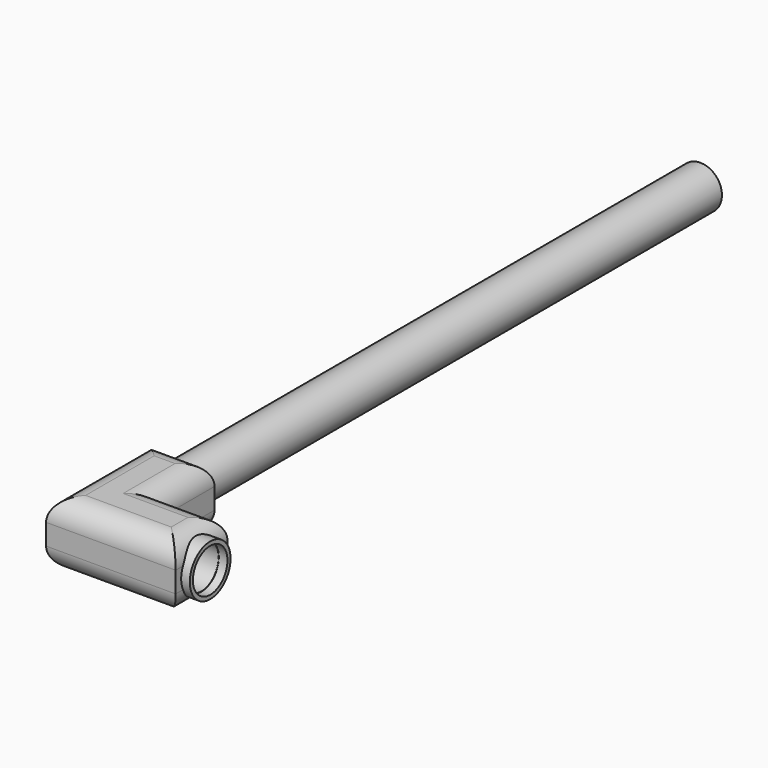
from build123d import *

# Parameters (mm, degrees)
F0_W          = 15
F0_H          = 15
F0_W_2        = 10
F0_H_2        = 10
F1_DEPTH      = 30
F2_W          = 15
F2_H          = 15
F2_W_2        = 10
F2_H_2        = 10
F4_DEPTH      = 15
F3_W          = 10
F3_H          = 10
F5_DEPTH      = 30
F6_R          = 5
F6_R_2        = 4.4707642424
F7_DEPTH      = 150
F8_W          = 10
F8_H          = 10
F9_DEPTH      = 15
F10_R         = 5.9
F10_R_2       = 5
F11_DEPTH     = 2
F12_R         = 4.929647133
F13_DEPTH     = 25.4
F14_T1_DEPTH  = 27.7
F14_T3_DEPTH  = 27.7
F14_T5_DEPTH  = 55.4
F14_T7_DEPTH  = 55.4
F14_T9_DEPTH  = 40.4
F14_T14_DEPTH = 40.4
F14_S15_R     = 5.9
F14_T16_DEPTH = 22
F14_T20_DEPTH = 40.4
F14_S21_R     = 5.9
F14_T22_DEPTH = 22
F14_T27_DEPTH = 27.7
F14_T31_DEPTH = 27.7
F14_S33_R     = 4.929647133
F14_T34_DEPTH = 16
F14_T40_DEPTH = 27.7
F14_T44_DEPTH = 27.7
F14_S46_R     = 4.929647133
F14_T47_DEPTH = 16


# Not quite as in the source:
# - a fillet or chamfer that OpenCascade refuses, or shapes differently, is made with other operations: its cross-section is extruded or revolved along the edge and cut away or added


with BuildPart() as f1:
    # F0 (on Front) → F1 (new body)
    with BuildSketch(Plane.XZ):
        Rectangle(F0_W, F0_H)
        Rectangle(F0_W_2, F0_H_2, mode=Mode.SUBTRACT)
    extrude(amount=F1_DEPTH)

    # F2 (on face) → F4 (join)
    with BuildSketch(Plane.YZ.offset(7.5)):
        with Locations((-22.5, 0)):
            Rectangle(F2_W, F2_H)
        with Locations((-22.5, 0)):
            Rectangle(F2_W_2, F2_H_2, mode=Mode.SUBTRACT)
    extrude(amount=F4_DEPTH)

    # F3 (on face) → F5 (join)
    with BuildSketch(Plane.XZ.offset(30)):
        Rectangle(F3_W, F3_H)
    extrude(amount=-F5_DEPTH)

    # F8 (on face) → F9 (join)
    with BuildSketch(Plane.YZ.offset(7.5)):
        with Locations((-22.5, 0)):
            Rectangle(F8_W, F8_H)
    extrude(amount=F9_DEPTH)

    # F10 (on face) → F11 (join)
    with BuildSketch(Plane.YZ.offset(22.5)):
        with Locations((-22.5, 0)):
            Circle(F10_R)
        with Locations((-22.5, 0)):
            Circle(F10_R_2, mode=Mode.SUBTRACT)
    extrude(amount=F11_DEPTH)

    # F12 (on face) → F13 (cut)
    with BuildSketch(Plane.YZ.offset(22.5)):
        with Locations((-22.5, 0)):
            Circle(F12_R)
    extrude(amount=-F13_DEPTH, mode=Mode.SUBTRACT)

    # F14: fillet of radius 5.08 on 12 edges, made by hand

    # F14_s2 → F14_t1 (cut)
    with BuildSketch(Plane.XZ.offset(-12.7)):
        with BuildLine():
            ThreePointArc((7.5, 2.42), (6.0121024484, 6.0121024484), (2.42, 7.5))
            Line((2.42, 7.5), (7.5, 7.5))
            Line((7.5, 7.5), (7.5, 2.42))
        make_face()
        with BuildLine():
            ThreePointArc((2.42, -7.5), (6.0121024484, -6.0121024484), (7.5, -2.42))
            Line((7.5, -2.42), (7.5, -7.5))
            Line((7.5, -7.5), (2.42, -7.5))
        make_face()
    extrude(amount=F14_T1_DEPTH, mode=Mode.SUBTRACT)

    # F14_s4 → F14_t3 (cut)
    with BuildSketch(Plane.YZ.offset(7.5)):
        with BuildLine():
            ThreePointArc((-15, 2.42), (-16.4878975516, 6.0121024484), (-20.08, 7.5))
            Line((-20.08, 7.5), (-15, 7.5))
            Line((-15, 7.5), (-15, 2.42))
        make_face()
        with BuildLine():
            ThreePointArc((-20.08, -7.5), (-16.4878975516, -6.0121024484), (-15, -2.42))
            Line((-15, -2.42), (-15, -7.5))
            Line((-15, -7.5), (-20.08, -7.5))
        make_face()
    extrude(amount=F14_T3_DEPTH, mode=Mode.SUBTRACT)

    # F14_s6 → F14_t5 (cut)
    with BuildSketch(Plane.YZ.offset(-20.2)):
        with BuildLine():
            ThreePointArc((-30, 2.42), (-28.5121024484, 6.0121024484), (-24.92, 7.5))
            Line((-24.92, 7.5), (-30, 7.5))
            Line((-30, 7.5), (-30, 2.42))
        make_face()
        with BuildLine():
            ThreePointArc((-24.92, -7.5), (-28.5121024484, -6.0121024484), (-30, -2.42))
            Line((-30, -2.42), (-30, -7.5))
            Line((-30, -7.5), (-24.92, -7.5))
        make_face()
    extrude(amount=F14_T5_DEPTH, mode=Mode.SUBTRACT)

    # F14_s8 → F14_t7 (cut)
    with BuildSketch(Plane.XZ.offset(-12.7)):
        with BuildLine():
            ThreePointArc((-7.5, 2.42), (-6.0121024484, 6.0121024484), (-2.42, 7.5))
            Line((-2.42, 7.5), (-7.5, 7.5))
            Line((-7.5, 7.5), (-7.5, 2.42))
        make_face()
        with BuildLine():
            ThreePointArc((-2.42, -7.5), (-6.0121024484, -6.0121024484), (-7.5, -2.42))
            Line((-7.5, -2.42), (-7.5, -7.5))
            Line((-7.5, -7.5), (-2.42, -7.5))
        make_face()
    extrude(amount=F14_T7_DEPTH, mode=Mode.SUBTRACT)

    # F14_s10 → F14_t9 (cut)
    with BuildSketch(Plane.YZ.offset(-20.2)):
        with BuildLine():
            ThreePointArc((0, 2.42), (-1.4878975516, 6.0121024484), (-5.08, 7.5))
            Line((-5.08, 7.5), (0, 7.5))
            Line((0, 7.5), (0, 2.42))
        make_face()
        with BuildLine():
            ThreePointArc((-5.08, -7.5), (-1.4878975516, -6.0121024484), (0, -2.42))
            Line((0, -2.42), (0, -7.5))
            Line((0, -7.5), (-5.08, -7.5))
        make_face()
    extrude(amount=F14_T9_DEPTH, mode=Mode.SUBTRACT)


with BuildPart() as f7:
    # F6 (on face) → F7 (new body)
    with BuildSketch(Plane(origin=(0, 0, 0), x_dir=(-1, 0, 0), z_dir=(0, 1, 0))):
        Circle(F6_R)
        Circle(F6_R_2, mode=Mode.SUBTRACT)
    extrude(amount=F7_DEPTH)


with BuildPart() as f14_tool12:
    # F14_s13 → F14_t14 (new body)
    with BuildSketch(Plane.XZ.offset(2.3)):
        with BuildLine():
            ThreePointArc((22.5, 2.42), (21.0121024484, 6.0121024484), (17.42, 7.5))
            Line((17.42, 7.5), (22.5, 7.5))
            Line((22.5, 7.5), (22.5, 2.42))
        make_face()
    extrude(amount=F14_T14_DEPTH)

    # F14_s15 → F14_t16 (cut, symmetric)
    with BuildSketch(Plane.YZ.offset(20)):
        with Locations((-22.5, 0)):
            Circle(F14_S15_R)
    extrude(amount=F14_T16_DEPTH, both=True, mode=Mode.SUBTRACT)


with BuildPart() as f1_1:
    add(f1.part)

    # F14_t11: cut F14_tool12
    add(f14_tool12.part, mode=Mode.SUBTRACT)


with BuildPart() as f14_tool18:
    # F14_s19 → F14_t20 (new body)
    with BuildSketch(Plane.XZ.offset(42.7)):
        with BuildLine():
            ThreePointArc((17.42, -7.5), (21.0121024484, -6.0121024484), (22.5, -2.42))
            Line((22.5, -2.42), (22.5, -7.5))
            Line((22.5, -7.5), (17.42, -7.5))
        make_face()
    extrude(amount=-F14_T20_DEPTH)

    # F14_s21 → F14_t22 (cut, symmetric)
    with BuildSketch(Plane.YZ.offset(20)):
        with Locations((-22.5, 0)):
            Circle(F14_S21_R)
    extrude(amount=F14_T22_DEPTH, both=True, mode=Mode.SUBTRACT)


with BuildPart() as f1_2:
    add(f1_1.part)

    # F14_t17: cut F14_tool18
    add(f14_tool18.part, mode=Mode.SUBTRACT)


with BuildPart() as f14_tool25:
    # F14_s26 → F14_t27 (new body)
    with BuildSketch(Plane.YZ.offset(-5.2)):
        with BuildLine():
            ThreePointArc((-15, 2.42), (-16.4878975516, 6.0121024484), (-20.08, 7.5))
            Line((-20.08, 7.5), (-15, 7.5))
            Line((-15, 7.5), (-15, 2.42))
        make_face()
    extrude(amount=F14_T27_DEPTH)

    split(bisect_by=Plane.YZ.offset(7.5), keep=Keep.BOTTOM)


with BuildPart() as f14_tool29:
    # F14_s30 → F14_t31 (new body)
    with BuildSketch(Plane.XZ):
        with BuildLine():
            ThreePointArc((7.5, 2.42), (6.0121024484, 6.0121024484), (2.42, 7.5))
            Line((2.42, 7.5), (7.5, 7.5))
            Line((7.5, 7.5), (7.5, 2.42))
        make_face()
    extrude(amount=F14_T31_DEPTH)

    split(bisect_by=Plane.XZ.offset(15), keep=Keep.TOP)

    # F14_s33 → F14_t34 (cut, symmetric)
    with BuildSketch(Plane.YZ.offset(5)):
        with Locations((-22.5, 0)):
            Circle(F14_S33_R)
    extrude(amount=F14_T34_DEPTH, both=True, mode=Mode.SUBTRACT)


with BuildPart() as f14_tool25_1:
    add(f14_tool25.part)

    # F14_t35: intersect F14_tool29
    add(f14_tool29.part, mode=Mode.INTERSECT)


with BuildPart() as f1_3:
    add(f1_2.part)

    # F14_t23: cut F14_tool25
    add(f14_tool25_1.part, mode=Mode.SUBTRACT)


with BuildPart() as f14_tool38:
    # F14_s39 → F14_t40 (new body)
    with BuildSketch(Plane.YZ.offset(-5.2)):
        with BuildLine():
            ThreePointArc((-20.08, -7.5), (-16.4878975516, -6.0121024484), (-15, -2.42))
            Line((-15, -2.42), (-15, -7.5))
            Line((-15, -7.5), (-20.08, -7.5))
        make_face()
    extrude(amount=F14_T40_DEPTH)

    split(bisect_by=Plane.YZ.offset(7.5), keep=Keep.BOTTOM)


with BuildPart() as f14_tool42:
    # F14_s43 → F14_t44 (new body)
    with BuildSketch(Plane.XZ):
        with BuildLine():
            ThreePointArc((2.42, -7.5), (6.0121024484, -6.0121024484), (7.5, -2.42))
            Line((7.5, -2.42), (7.5, -7.5))
            Line((7.5, -7.5), (2.42, -7.5))
        make_face()
    extrude(amount=F14_T44_DEPTH)

    split(bisect_by=Plane.XZ.offset(15), keep=Keep.TOP)

    # F14_s46 → F14_t47 (cut, symmetric)
    with BuildSketch(Plane.YZ.offset(5)):
        with Locations((-22.5, 0)):
            Circle(F14_S46_R)
    extrude(amount=F14_T47_DEPTH, both=True, mode=Mode.SUBTRACT)


with BuildPart() as f14_tool38_1:
    add(f14_tool38.part)

    # F14_t48: intersect F14_tool42
    add(f14_tool42.part, mode=Mode.INTERSECT)


with BuildPart() as f1_4:
    add(f1_3.part)

    # F14_t36: cut F14_tool38
    add(f14_tool38_1.part, mode=Mode.SUBTRACT)


solid = Compound([f7.part, f1_4.part])
